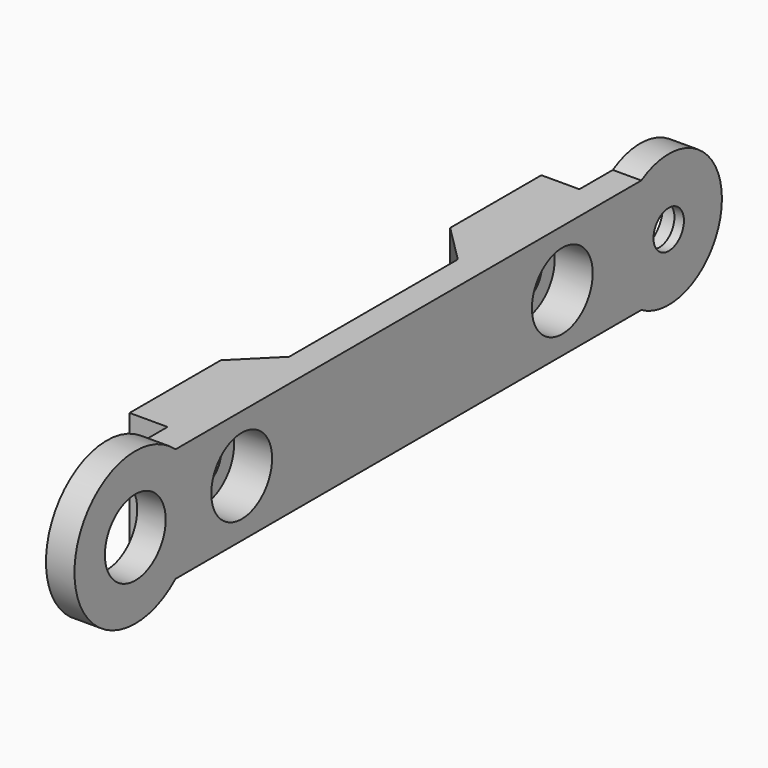
from build123d import *

# Parameters (mm, degrees)
F1_DEPTH  = 9.525
F2_R      = 5.55625
F2_R_2    = 6.35
F3_DEPTH  = 2.38125
F4_R      = 3.175
F4_R_2    = 1.8288
F4_R_3    = 1.5875
F5_DEPTH  = 5.55625
F6_R      = 2.38125
F7_DEPTH  = 1.5875
F8_SIZE   = 3.17499
F9_R      = 3.175
F10_DEPTH = 3.175


# Not quite as in the source:
# - a fillet or chamfer is up to 0.001 mm smaller than in the source, because OpenCascade refuses the exact size


with BuildPart() as f1:
    # F0 (on Top) → F1 (new body)
    with BuildSketch(Plane.XY):
        Polygon((0, 0), (0, 55.7060608), (-2.38125, 55.7060608), (-2.38125, 49.3560608), (-5.55625, 49.3560608), (-5.55625, 39.8310608), (-2.38125, 39.8310608), (-2.38125, 15.875), (-5.55625, 15.875), (-5.55625, 6.35), (-2.38125, 6.35), (-2.38125, 0), align=None)
    extrude(amount=F1_DEPTH)

    # F2 (on face) → F3 (join, through all)
    with BuildSketch(Plane(origin=(-2.38125, 0, 0), x_dir=(0, -1, 0), z_dir=(-1, 0, 0))):
        with Locations((-55.7060608, 4.7625)):
            Circle(F2_R)
        with Locations((0, 4.7625)):
            Circle(F2_R_2)
    extrude(amount=-F3_DEPTH)

    # F4 (on face) → F5 (cut, through all)
    with BuildSketch(Plane.YZ):
        with Locations((0, 4.7625)):
            Circle(F4_R)
        with Locations((11.1125, 4.7625)):
            Circle(F4_R_2)
        with Locations((44.5935608, 4.7625)):
            Circle(F4_R_2)
        with Locations((55.7060608001, 4.7625)):
            Circle(F4_R_3)
    extrude(amount=-F5_DEPTH, mode=Mode.SUBTRACT)

    # F6 (on face) → F7 (cut)
    with BuildSketch(Plane(origin=(-2.38125, 0, 0), x_dir=(0, -1, 0), z_dir=(-1, 0, 0))):
        with Locations((-55.7060608, 4.7625)):
            Circle(F6_R)
    extrude(amount=-F7_DEPTH, mode=Mode.SUBTRACT)

    # F8 (size 3.175 in the source; OpenCascade refuses exactly that, so slightly less here)
    f8_edges = [f1.edges().sort_by_distance(p)[0] for p in [
        (-2.38125, 39.831061, 4.7625),
        (-2.38125, 15.875, 4.7625),
    ]]
    chamfer(f8_edges, length=F8_SIZE)

    # F9 (on face) → F10 (cut)
    with BuildSketch(Plane.YZ):
        with Locations((11.1125, 4.7625)):
            Circle(F9_R)
        with Locations((44.5935608, 4.7625)):
            Circle(F9_R)
    extrude(amount=-F10_DEPTH, mode=Mode.SUBTRACT)


solid = f1.part
